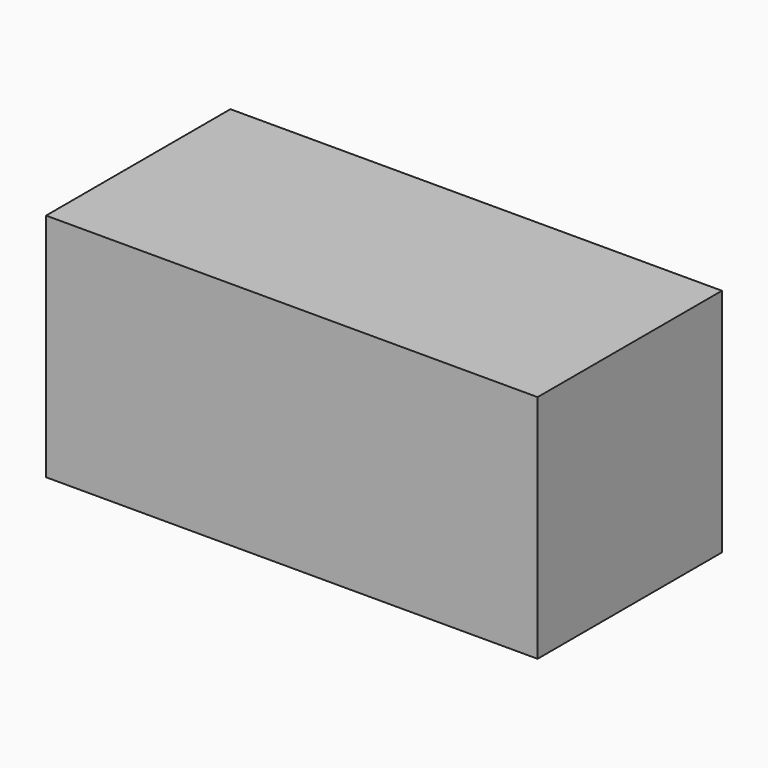
from build123d import *

# Parameters (mm, degrees)
F0_W     = 40
F0_H     = 15
F1_DEPTH = 15
F2_W     = 14
F2_H     = 14
F3_DEPTH = 15
F4_R     = 6.99999
F5_DEPTH = 8


# Not quite as in the source:
# - a fillet or chamfer is up to 0.001 mm smaller than in the source, because OpenCascade refuses the exact size


with BuildPart() as f1:
    # F0 (on Top) → F1 (new body)
    with BuildSketch(Plane.XY):
        with Locations((20, 7.5)):
            Rectangle(F0_W, F0_H)
    extrude(amount=F1_DEPTH)

    # F2 (on face) → F3 (cut)
    with BuildSketch(Plane(origin=(0, 0, 0), x_dir=(0, -1, 0), z_dir=(-1, 0, 0))):
        with Locations((-7.5, 7.5)):
            Rectangle(F2_W, F2_H)
    extrude(amount=-F3_DEPTH, mode=Mode.SUBTRACT)

    # F4 (radius 7 in the source; OpenCascade refuses exactly that, so slightly less here)
    f4_edges = [f1.edges().sort_by_distance(p)[0] for p in [
        (15, 7.5, 14.5),
        (15, 14.5, 7.5),
        (7.5, 14.5, 14.5),
        (15, 0.5, 7.5),
        (15, 7.5, 0.5),
        (7.5, 0.5, 14.5),
        (7.5, 0.5, 0.5),
        (7.5, 14.5, 0.5),
    ]]
    fillet(f4_edges, radius=F4_R)

    # F5 (cut): a face of the model
    f5_faces = [f1.faces().sort_by_distance(p)[0] for p in [
        (0, 0.2878679656, 7.5),
    ]]
    extrude(f5_faces, amount=-F5_DEPTH, mode=Mode.SUBTRACT)


solid = f1.part
